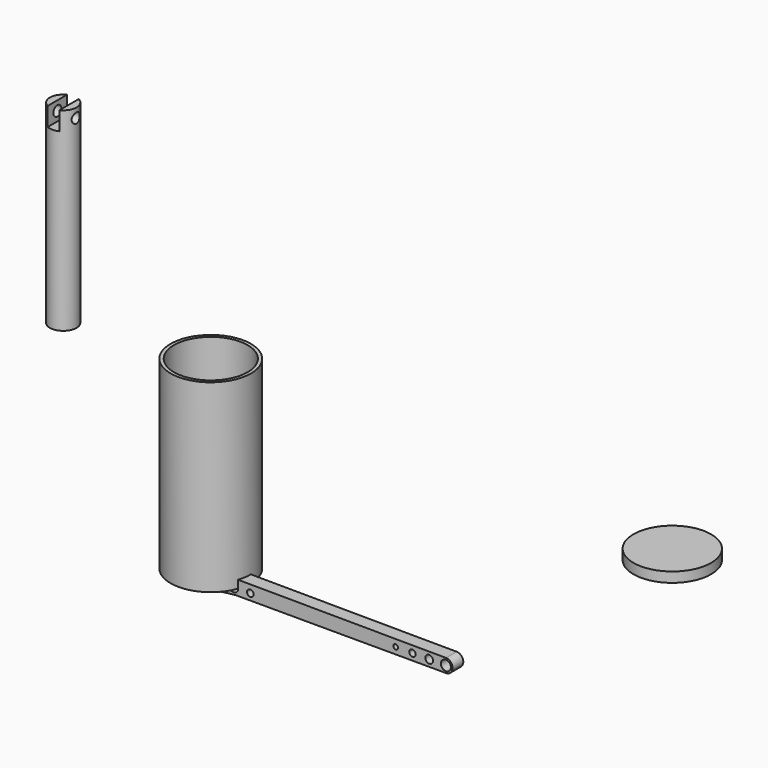
from build123d import *

# Parameters (mm, degrees)
F2_R      = 5.8
F3_DEPTH  = 1.5
F4_R      = 2
F5_DEPTH  = 29
F7_DEPTH  = 2.78
F0_R      = 6
F8_DEPTH  = 27.6
F9_R      = 5.5
F10_DEPTH = 27.6
F11_R     = 1
F11_R_2   = 0.8560808417
F11_R_3   = 0.6939243984
F11_R_4   = 0.4925851038
F11_R_5   = 0.3563326194
F11_R_6   = 0.4777702974
F11_R_7   = 0.5835711178
F11_R_8   = 0.75
F12_DEPTH = 2
F13_R     = 0.75
F14_DEPTH = 4
F15_R     = 0.75
F16_DEPTH = 54.1968321333


# Not quite as in the source:
# - the program builds the solid bodies; features that only make, move or delete a surface that nothing else refers to are left out


with BuildPart() as f3:
    # F2 (on Top) → F3 (new body)
    with BuildSketch(Plane.XY):
        with Locations((40.6981445849, 35.3143140674)):
            Circle(F2_R)
    extrude(amount=F3_DEPTH)


with BuildPart() as f5:
    # F4 (on Top) → F5 (new body)
    with BuildSketch(Plane.XY):
        with Locations((-52.1958321333, 37.6868508756)):
            Circle(F4_R)
    extrude(amount=F5_DEPTH)

    # F6 (on face) → F7 (cut)
    with BuildSketch(Plane.XY.offset(29)):
        with BuildLine():
            ThreePointArc((-51.3208321333, 39.4852876969), (-52.1958321333, 39.6868508756), (-53.0708321333, 39.4852876969))
            Line((-53.0708321333, 39.4852876969), (-53.0708321333, 35.8884140544))
            ThreePointArc((-53.0708321333, 35.8884140544), (-52.1958321333, 35.6868508756), (-51.3208321333, 35.8884140544))
            Line((-51.3208321333, 35.8884140544), (-51.3208321333, 39.4852876969))
        make_face()
    extrude(amount=-F7_DEPTH, mode=Mode.SUBTRACT)

    # F15 (on Right) → F16 (cut, through all)
    with BuildSketch(Plane.YZ):
        with Locations((37.6869140544, 27.61)):
            Circle(F15_R)
    extrude(amount=-F16_DEPTH, mode=Mode.SUBTRACT)


with BuildPart() as f8:
    # F0 (on Top) → F8 (new body)
    with BuildSketch(Plane.XY):
        Circle(F0_R)
    extrude(amount=F8_DEPTH)

    # F9 (on face) → F10 (cut)
    with BuildSketch(Plane.XY.offset(27.6)):
        Circle(F9_R)
    extrude(amount=-F10_DEPTH, mode=Mode.SUBTRACT)


with BuildPart() as f12:
    # F11 (on Front) → F12 (new body)
    with BuildSketch(Plane.XZ):
        with BuildLine():
            ThreePointArc((5.169888125, 1.1790200467), (2.5774452808, 1.4107420589), (0, 1.773))
            ThreePointArc((0, 1.773), (-1.773, 0), (0, -1.773))
            ThreePointArc((0, -1.773), (2.6128788251, -1.3020949548), (5.2465344779, -0.9663194069))
            Line((5.2465344779, -0.9663194069), (36.6588703738, -0.9976764776))
            ThreePointArc((36.6588703738, -0.9976764776), (37.7263182617, -0.0369189891), (36.7326722897, 0.9999839124))
            Line((36.7326722897, 0.9999839124), (5.169888125, 1.1790200467))
        make_face()
        Circle(F11_R, mode=Mode.SUBTRACT)
        with Locations((2.5, 0)):
            Circle(F11_R_2, mode=Mode.SUBTRACT)
        with Locations((5, 0)):
            Circle(F11_R_3, mode=Mode.SUBTRACT)
        with Locations((7.5, 0)):
            Circle(F11_R_4, mode=Mode.SUBTRACT)
        with Locations((29.227, 0)):
            Circle(F11_R_5, mode=Mode.SUBTRACT)
        with Locations((31.727, 0)):
            Circle(F11_R_6, mode=Mode.SUBTRACT)
        with Locations((34.227, 0)):
            Circle(F11_R_7, mode=Mode.SUBTRACT)
        with Locations((36.727, 0)):
            Circle(F11_R_8, mode=Mode.SUBTRACT)
    extrude(amount=F12_DEPTH)


with BuildPart() as f14:
    # F13 (on Right) → F14 (new body)
    with BuildSketch(Plane.YZ):
        Circle(F13_R)
    extrude(amount=F14_DEPTH)


solid = Compound([f3.part, f5.part, f8.part, f12.part, f14.part])
